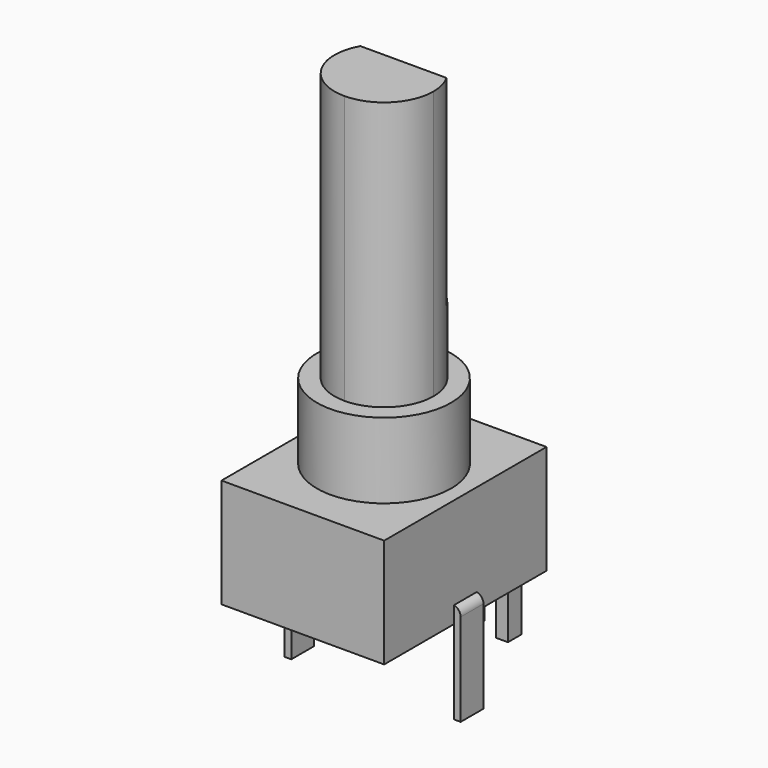
from build123d import *

# Parameters (mm, degrees)
F0_W         = 9.7
F0_H         = 12.1
F0_R         = 4
F1_DEPTH     = 6.5
F2_DEPTH     = 4.5
F4_DEPTH     = 16
F5_DEPTH     = 4
F6_W         = 0.7
F6_H         = 4.5
F6_H_2       = 1
F6_W_2       = 0.35
F7_DEPTH     = 1
F8_R         = 0.99999
F9_W         = 0.85
F9_H         = 1
F10_DEPTH    = 0.4
F11_T1_DEPTH = 4.1494897428
F12_W        = 0.85
F12_H        = 1
F13_DEPTH    = 0.4
F14_T1_DEPTH = 4.1494897428


# Not quite as in the source:
# - a fillet or chamfer that OpenCascade refuses, or shapes differently, is made with other operations: its cross-section is extruded or revolved along the edge and cut away or added
# - a fillet or chamfer is up to 0.001 mm smaller than in the source, because OpenCascade refuses the exact size


with BuildPart() as f1:
    # F0 (on Top) → F1 (new body)
    with BuildSketch(Plane.XY):
        with Locations((-29.8902173527, 8.9015606931)):
            Rectangle(F0_W, F0_H)
        with Locations((-29.8902173527, 8.9015606931)):
            Circle(F0_R, mode=Mode.SUBTRACT)
        with Locations((-29.8902173527, 8.9015606931)):
            Circle(F0_R)
    extrude(amount=-F1_DEPTH)

    # F0 (on Top) → F2 (join)
    with BuildSketch(Plane.XY):
        with Locations((-29.8902173527, 8.9015606931)):
            Circle(F0_R)
    extrude(amount=F2_DEPTH)

    # F3 (on face) → F4 (join)
    with BuildSketch(Plane.XY.offset(4.5)):
        with BuildLine():
            ThreePointArc((-32.4592638684, 10.3515606931), (-32.4377651932, 7.4141132151), (-29.8902173527, 5.9515606931))
            Line((-29.8902173527, 5.9515606931), (-29.8902173527, 10.3515606931))
            Line((-29.8902173527, 10.3515606931), (-32.4592638684, 10.3515606931))
        make_face()
        with BuildLine():
            ThreePointArc((-29.8902173527, 5.9515606931), (-27.8042523482, 6.8155956886), (-26.9402173527, 8.9015606931))
            ThreePointArc((-26.9402173527, 8.9015606931), (-27.0370448008, 9.6511648482), (-27.3211708369, 10.3515606931))
            Line((-27.3211708369, 10.3515606931), (-29.8902173527, 10.3515606931))
            Line((-29.8902173527, 10.3515606931), (-29.8902173527, 5.9515606931))
        make_face()
    extrude(amount=F4_DEPTH)

    # F3 (on face) → F5 (join)
    with BuildSketch(Plane.XY.offset(4.5)):
        with BuildLine():
            Line((-29.8902173527, 10.3515606931), (-27.3211708369, 10.3515606931))
            ThreePointArc((-27.3211708369, 10.3515606931), (-29.8902173527, 11.8515606931), (-32.4592638684, 10.3515606931))
            Line((-32.4592638684, 10.3515606931), (-29.8902173527, 10.3515606931))
        make_face()
    extrude(amount=F5_DEPTH)

    # F6 (on face) → F7 (join)
    with BuildSketch(Plane(origin=(0, 14.9515606931, 0), x_dir=(-1, 0, 0), z_dir=(0, 1, 0))):
        with Locations((27.6902173527, -8.75)):
            Rectangle(F6_W, F6_H)
        with Locations((27.6902173527, -6)):
            Rectangle(F6_W, F6_H_2)
        with Locations((29.7152173527, -6)):
            Rectangle(F6_W_2, F6_H_2)
        with Locations((30.0652173527, -6)):
            Rectangle(F6_W_2, F6_H_2)
        Polygon((30.2402173527, -11), (30.2402173527, -6.5), (29.8902173527, -6.5), (29.5402173527, -6.5), (29.5402173527, -11), align=None)
        with Locations((32.0902173527, -6)):
            Rectangle(F6_W, F6_H_2)
        with Locations((32.0902173527, -8.75)):
            Rectangle(F6_W, F6_H)
    extrude(amount=F7_DEPTH)

    # F8 (radius 1 in the source; OpenCascade refuses exactly that, so slightly less here)
    f8_edges = [f1.edges().sort_by_distance(p)[0] for p in [
        (-27.690217, 15.951561, -5.5),
        (-29.890217, 15.951561, -5.5),
        (-32.090217, 15.951561, -5.5),
    ]]
    fillet(f8_edges, radius=F8_R)

    # F9 (on face) → F10 (join)
    with BuildSketch(Plane.YZ.offset(-25.0402173527)):
        with Locations((8.4765606931, -6)):
            Rectangle(F9_W, F9_H)
        with Locations((9.3265606931, -6)):
            Rectangle(F9_W, F9_H)
        Polygon((9.7515606931, -6.5), (8.9015606931, -6.5), (8.0515606931, -6.5), (8.0515606931, -11.5), (9.7515606931, -11.5), align=None)
    extrude(amount=F10_DEPTH)

    # F11: fillet of radius 0.5 on 1 edges, made by hand

    # F11_s2 → F11_t1 (cut)
    with BuildSketch(Plane.XZ.offset(-10.9763055645)):
        with BuildLine():
            ThreePointArc((-25.0402173527, -5.5), (-24.752919018, -5.6736701825), (-24.6402173527, -5.9898979486))
            Line((-24.6402173527, -5.9898979486), (-24.6402173527, -5.5))
            Line((-24.6402173527, -5.5), (-25.0402173527, -5.5))
        make_face()
    extrude(amount=F11_T1_DEPTH, mode=Mode.SUBTRACT)

    # F12 (on face) → F13 (join)
    with BuildSketch(Plane(origin=(-34.7402173527, 0, 0), x_dir=(0, -1, 0), z_dir=(-1, 0, 0))):
        with Locations((-9.3265606931, -6)):
            Rectangle(F12_W, F12_H)
        with Locations((-8.4765606931, -6)):
            Rectangle(F12_W, F12_H)
        Polygon((-8.9015606931, -6.5), (-9.7515606931, -6.5), (-9.7515606931, -11.5), (-8.0515606931, -11.5), (-8.0515606931, -6.5), align=None)
    extrude(amount=F13_DEPTH)

    # F14: fillet of radius 0.5 on 1 edges, made by hand

    # F14_s2 → F14_t1 (cut)
    with BuildSketch(Plane.XZ.offset(-10.9763055645)):
        with BuildLine():
            ThreePointArc((-34.7402173527, -5.5), (-35.0275156873, -5.6736701825), (-35.1402173527, -5.9898979486))
            Line((-35.1402173527, -5.9898979486), (-35.1402173527, -5.5))
            Line((-35.1402173527, -5.5), (-34.7402173527, -5.5))
        make_face()
    extrude(amount=F14_T1_DEPTH, mode=Mode.SUBTRACT)


solid = f1.part
